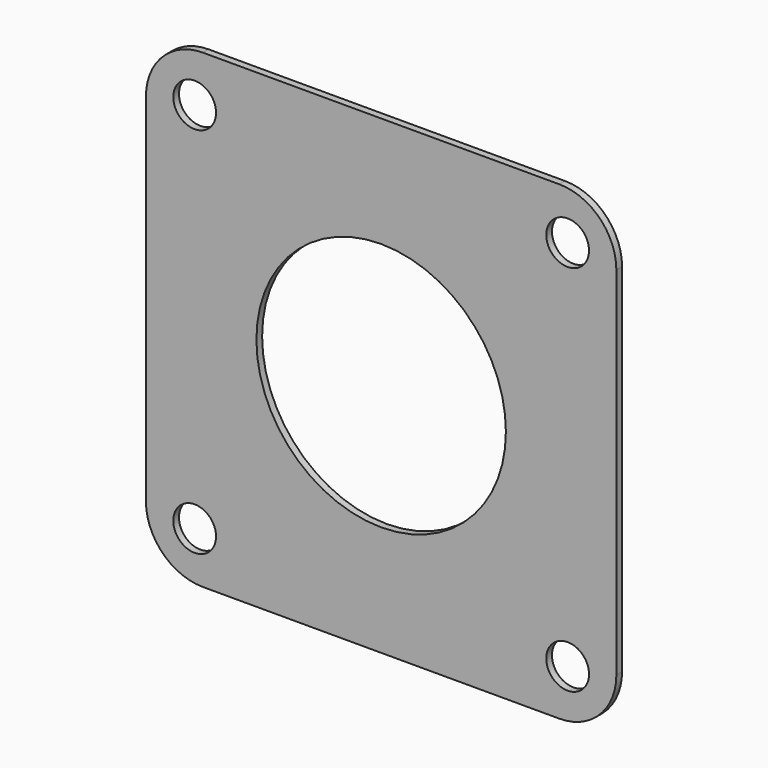
from build123d import *

# Parameters (mm, degrees)
F0_R     = 4.7625
F0_R_2   = 27.78125
F1_DEPTH = 1.5875


# Not quite as in the source:
# - a length typed as a fraction of an inch, garbled in the dataset ("3 / 203.2 mm" for 3/8 in), is restored


with BuildPart() as f1:
    # F0 (on Front) → F1 (new body)
    with BuildSketch(Plane.XZ):
        with BuildLine():
            ThreePointArc((0, 12.7), (3.7197438789, 3.7197438789), (12.7, 0))
            Line((12.7, 0), (92.075, 0))
            ThreePointArc((92.075, 0), (101.0552561211, 3.7197438789), (104.775, 12.7))
            Line((104.775, 12.7), (104.775, 92.075))
            ThreePointArc((104.775, 92.075), (101.0552561211, 101.0552561211), (92.075, 104.775))
            Line((92.075, 104.775), (12.7, 104.775))
            ThreePointArc((12.7, 104.775), (3.7197438789, 101.0552561211), (0, 92.075))
            Line((0, 92.075), (0, 12.7))
        make_face()
        with Locations((10.8538154401, 10.8538154401)):
            Circle(F0_R, mode=Mode.SUBTRACT)
        with Locations((93.9211845599, 10.8538154401)):
            Circle(F0_R, mode=Mode.SUBTRACT)
        with Locations((10.8538154401, 93.9211845599)):
            Circle(F0_R, mode=Mode.SUBTRACT)
        with Locations((52.3875, 52.3875)):
            Circle(F0_R_2, mode=Mode.SUBTRACT)
        with Locations((93.9211845599, 93.9211845599)):
            Circle(F0_R, mode=Mode.SUBTRACT)
    extrude(amount=F1_DEPTH)


solid = f1.part
